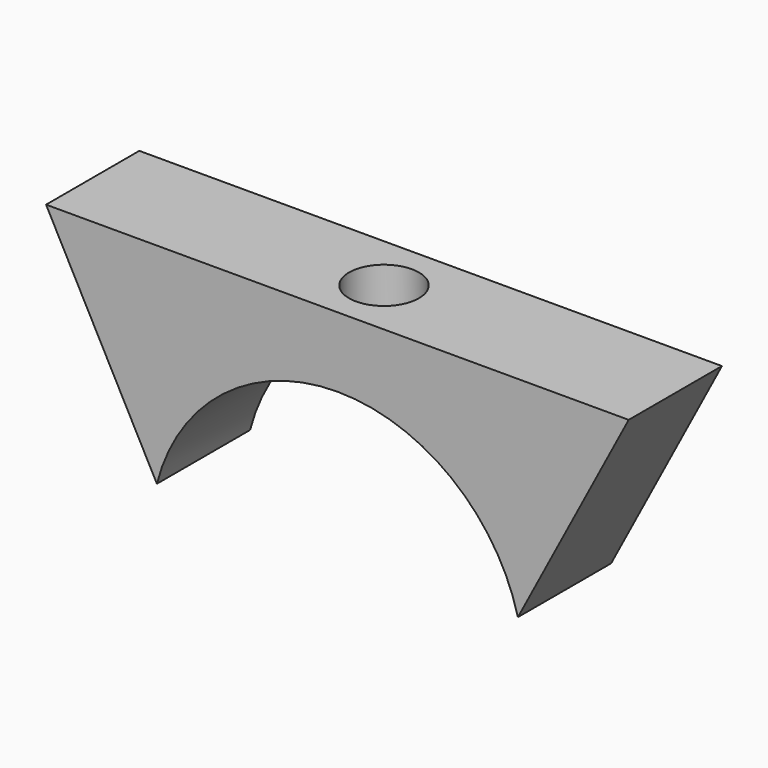
from build123d import *

# Parameters (mm, degrees)
F1_DEPTH = 2.5
F2_R     = 1.5
F3_DEPTH = 11.001


# Not quite as in the source:
# - a feature names something its author has since deleted; it is built from what else it names


with BuildPart() as f1:
    # F0 (on Front) → F1 (new body, symmetric)
    with BuildSketch(Plane.XZ):
        with BuildLine():
            Line((12.5, 11), (-12.5, 11))
            Line((-12.5, 11), (-7.7459666924, 2))
            ThreePointArc((-7.7459666924, 2), (0, 8), (7.7459666924, 2))
            Line((7.7459666924, 2), (12.5, 11))
        make_face()
    extrude(amount=F1_DEPTH, both=True)

    # F2 (on Top) → F3 (cut, through all)
    with BuildSketch(Plane.XY):
        Circle(F2_R)
    extrude(amount=F3_DEPTH, mode=Mode.SUBTRACT)


solid = f1.part
